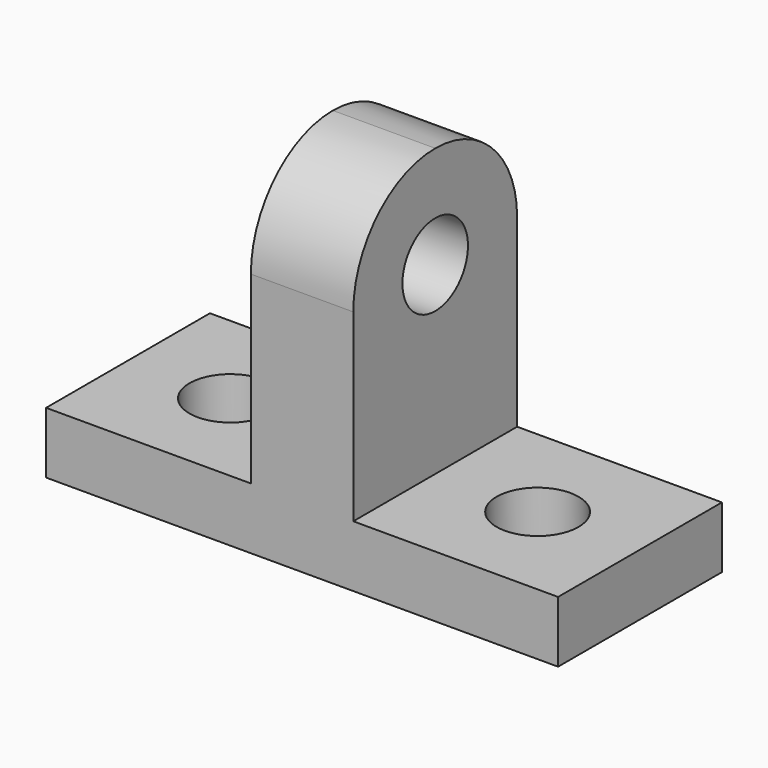
from build123d import *

# Parameters (mm, degrees)
F0_W     = 25
F0_H     = 10
F1_DEPTH = 3
F2_W     = 5
F2_H     = 10
F3_DEPTH = 14
F5_R     = 4.99999
F4_R     = 2
F7_DEPTH = 3
F6_R     = 2
F8_DEPTH = 5


# Not quite as in the source:
# - a fillet or chamfer is up to 0.001 mm smaller than in the source, because OpenCascade refuses the exact size


with BuildPart() as f1:
    # F0 (on Top) → F1 (new body)
    with BuildSketch(Plane.XY):
        with Locations((-42.0921362936, -7.1861277148)):
            Rectangle(F0_W, F0_H)
    extrude(amount=F1_DEPTH)

    # F2 (on face) → F3 (join)
    with BuildSketch(Plane.XY.offset(3)):
        with Locations((-42.0921362936, -7.1861277148)):
            Rectangle(F2_W, F2_H)
    extrude(amount=F3_DEPTH)

    # F5 (radius 5 in the source; OpenCascade refuses exactly that, so slightly less here)
    f5_edges = [f1.edges().sort_by_distance(p)[0] for p in [
        (-42.092136, -12.186128, 17),
        (-42.092136, -2.186128, 17),
    ]]
    fillet(f5_edges, radius=F5_R)

    # F4 (on face) → F7 (cut)
    with BuildSketch(Plane.XY.offset(3)):
        with Locations((-49.5921362936, -7.1861277148)):
            Circle(F4_R)
        with Locations((-34.5921362936, -7.1861277148)):
            Circle(F4_R)
    extrude(amount=-F7_DEPTH, mode=Mode.SUBTRACT)

    # F6 (on face) → F8 (cut)
    with BuildSketch(Plane(origin=(-44.5921362936, 0, 0), x_dir=(0, -1, 0), z_dir=(-1, 0, 0))):
        with Locations((7.1861277148, 12)):
            Circle(F6_R)
    extrude(amount=-F8_DEPTH, mode=Mode.SUBTRACT)


solid = f1.part
